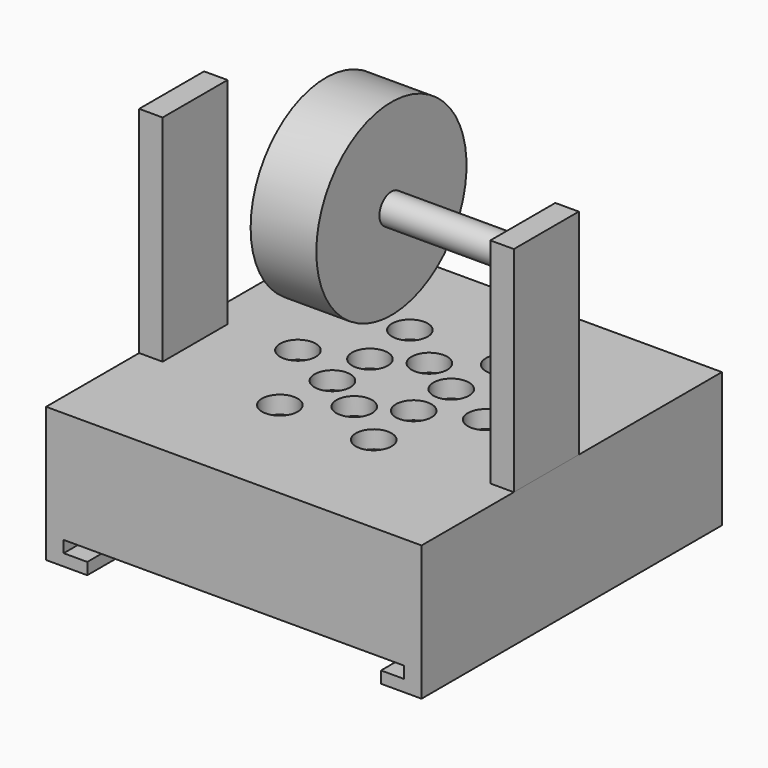
from build123d import *

# Parameters (mm, degrees)
F0_W      = 101.6
F0_H      = 101.6
F1_DEPTH  = 30.1625
F2_W      = 21.9635302201
F2_H      = 57.9157359898
F3_DEPTH  = 6.35
F4_W      = 21.9635302201
F4_H      = 58.17720294
F5_DEPTH  = 6.35
F7_T      = -4.7625
F6_R      = 4.826
F8_DEPTH  = 65.532
F9_W      = 4.7625
F9_H      = 101.6
F10_DEPTH = 6.35
F11_W     = 6.3828786112
F11_H     = 3.1750000536
F11_W_2   = 6.2050602607
F12_DEPTH = 101.6
F15_R     = 4.064
F16_DEPTH = 35.56
F17_R     = 25.4
F17_R_2   = 4.064
F18_DEPTH = 17.78


# Not quite as in the source:
# - the program builds the solid bodies; features that only make, move or delete a surface that nothing else refers to are left out


with BuildPart() as f1:
    # F0 (on Top) → F1 (new body)
    with BuildSketch(Plane.XY):
        with Locations((-57.7274323441, 8.9923822479)):
            Rectangle(F0_W, F0_H)
    extrude(amount=-F1_DEPTH)

    # F7
    f7_openings = [f1.faces().sort_by_distance(p)[0] for p in [
        (-57.727432, 8.992382, -30.1625),
    ]]
    offset(amount=F7_T, openings=f7_openings)

    # F6 (on face) → F8 (cut)
    with BuildSketch(Plane.XY):
        with Locations((-70.4274323441, 33.6324865892)):
            Circle(F6_R)
        with BuildLine():
            ThreePointArc((-40.2014323441, 33.6324865892), (-45.0274323441, 38.4584865892), (-49.8534323441, 33.6324865892))
            ThreePointArc((-49.8534323441, 33.6324865892), (-45.0274323441, 28.8064865892), (-40.2014323441, 33.6324865892))
        make_face()
        with Locations((-57.7274323441, 24.3354413331)):
            Circle(F6_R)
        with Locations((-46.728909716, 17.9854413331)):
            Circle(F6_R)
        with Locations((-46.728909716, 5.2854413331)):
            Circle(F6_R)
        with Locations((-32.3274323441, 11.6354413331)):
            Circle(F6_R)
        with Locations((-45.0274323441, -10.3616039231)):
            Circle(F6_R)
        with Locations((-57.7274323441, -1.0645586669)):
            Circle(F6_R)
        with Locations((-70.4274323441, -10.3616039231)):
            Circle(F6_R)
        with Locations((-68.7259549722, 5.2854413331)):
            Circle(F6_R)
        with Locations((-68.7259549722, 17.9854413331)):
            Circle(F6_R)
        with Locations((-83.1274323441, 11.6354413331)):
            Circle(F6_R)
    extrude(amount=-F8_DEPTH, mode=Mode.SUBTRACT)

    # F9 (on face) → F10 (join)
    with BuildSketch(Plane(origin=(0, 0, -30.1625), x_dir=(1, 0, 0), z_dir=(0, 0, -1))):
        with Locations((-106.1461823441, -8.9923822479)):
            Rectangle(F9_W, F9_H)
        with Locations((-9.3086823441, -8.9923822479)):
            Rectangle(F9_W, F9_H)
    extrude(amount=F10_DEPTH)

    # F11 (on face) → F12 (join)
    with BuildSketch(Plane.XZ.offset(41.8076177521)):
        with Locations((-100.5734930385, -34.9249999732)):
            Rectangle(F11_W, F11_H)
        with Locations((-14.7924624745, -34.9249999732)):
            Rectangle(F11_W_2, F11_H)
    extrude(amount=-F12_DEPTH)


with BuildPart() as f3:
    # F2 (on face) → F3 (new body)
    with BuildSketch(Plane.YZ.offset(-6.9274323441)):
        with Locations((0.3922064789, 28.9578679949)):
            Rectangle(F2_W, F2_H)
    extrude(amount=-F3_DEPTH)

    # F15 (on face) → F16 (join)
    with BuildSketch(Plane(origin=(-13.2774323441, 0, 0), x_dir=(0, -1, 0), z_dir=(-1, 0, 0))):
        with Locations((-0.3922064789, 49.4577102363)):
            Circle(F15_R)
    extrude(amount=F16_DEPTH)


with BuildPart() as f5:
    # F4 (on face) → F5 (new body)
    with BuildSketch(Plane(origin=(-108.5274323441, 0, 0), x_dir=(0, -1, 0), z_dir=(-1, 0, 0))):
        with Locations((-0.653676223, 29.08860147)):
            Rectangle(F4_W, F4_H)
    extrude(amount=-F5_DEPTH)


with BuildPart() as f18:
    # F17 (on face) → F18 (new body)
    with BuildSketch(Plane(origin=(-48.8374323441, 0, 0), x_dir=(0, -1, 0), z_dir=(-1, 0, 0))):
        with Locations((-0.3922064789, 49.4577102363)):
            Circle(F17_R)
        with Locations((-0.3922064789, 49.4577102363)):
            Circle(F17_R_2, mode=Mode.SUBTRACT)
    extrude(amount=F18_DEPTH)


solid = Compound([f1.part, f3.part, f5.part, f18.part])
